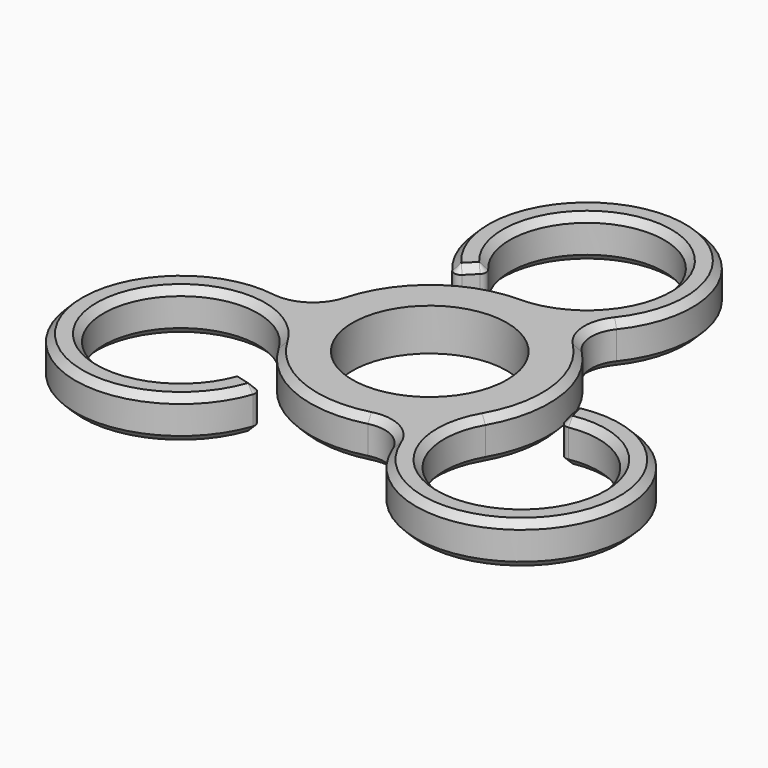
from build123d import *

# Parameters (mm, degrees)
F0_R     = 11
F1_DEPTH = 6
F2_SIZE  = 0.99999


# Not quite as in the source:
# - a fillet or chamfer is up to 0.001 mm smaller than in the source, because OpenCascade refuses the exact size


with BuildPart() as f1:
    # F0 (on Top) → F1 (new body)
    with BuildSketch(Plane.XY):
        with BuildLine():
            ThreePointArc((-8.3993012068, 20.8970612253), (4.6296691825, 37.9782845851), (0, 17))
            ThreePointArc((0, 17), (-10.3245446798, 13.5056942492), (-16.4047227892, 4.4592679005))
            ThreePointArc((-16.4047227892, 4.4592679005), (-18.5023983731, 1.580095835), (-21.984408769, 0.8281129622))
            ThreePointArc((-21.984408769, 0.8281129622), (-37.0912454672, -21.75043975), (-10.0741387442, -18.90728975))
            ThreePointArc((-10.0741387442, -18.90728975), (-10.1357694828, -18.1114057356), (-10.7602912032, -17.6142112737))
            Line((-10.7602912032, -17.6142112737), (-12.6979184167, -17.0950256266))
            ThreePointArc((-12.6979184167, -17.0950256266), (-13.420186678, -17.1748279717), (-13.8977352822, -17.7225388318))
            ThreePointArc((-13.8977352822, -17.7225388318), (-35.2049938341, -14.9797311694), (-14.7224318643, -8.5))
            ThreePointArc((-14.7224318643, -8.5), (-6.5340019757, -15.6941650999), (4.3405221105, -16.4365406278))
            ThreePointArc((4.3405221105, -16.4365406278), (7.882796053, -16.8135949396), (10.275037522, -19.4531129622))
            ThreePointArc((10.275037522, -19.4531129622), (37.3820561006, -21.2467409576), (21.4112626123, 0.7291848013))
            ThreePointArc((21.4112626123, 0.7291848013), (20.7528222067, 0.2778690088), (20.6345000323, -0.5115798972))
            Line((20.6345000323, -0.5115798972), (21.1536856793, -2.4492071107))
            ThreePointArc((21.1536856793, -2.4492071107), (21.5839306681, -3.0348086009), (22.297036489, -3.1745223935))
            ThreePointArc((22.297036489, -3.1745223935), (30.5753246516, -22.9985534157), (14.7224318643, -8.5))
            ThreePointArc((14.7224318643, -8.5), (16.8585466555, 2.1884708506), (12.0642006787, 11.9772727273))
            ThreePointArc((12.0642006787, 11.9772727273), (10.6196023201, 15.2334991046), (11.709371247, 18.625))
            ThreePointArc((11.709371247, 18.625), (-0.2908106334, 42.9971807076), (-11.3371238681, 18.1781049487))
            ThreePointArc((-11.3371238681, 18.1781049487), (-10.6170527239, 17.8335367268), (-9.8742088291, 18.1257911709))
            Line((-9.8742088291, 18.1257911709), (-8.4557672626, 19.5442327374))
            ThreePointArc((-8.4557672626, 19.5442327374), (-8.1637439901, 20.2096365726), (-8.3993012068, 20.8970612253))
        make_face()
        Circle(F0_R, mode=Mode.SUBTRACT)
    extrude(amount=F1_DEPTH)

    # F2 (size 1 in the source; OpenCascade refuses exactly that, so slightly less here)
    f2_edges = [f1.edges().sort_by_distance(p)[0] for p in [
        (-37.091245, -21.75044, 6),
        (37.382056, -21.246741, 0),
    ]]
    chamfer(f2_edges, length=F2_SIZE)


solid = f1.part
